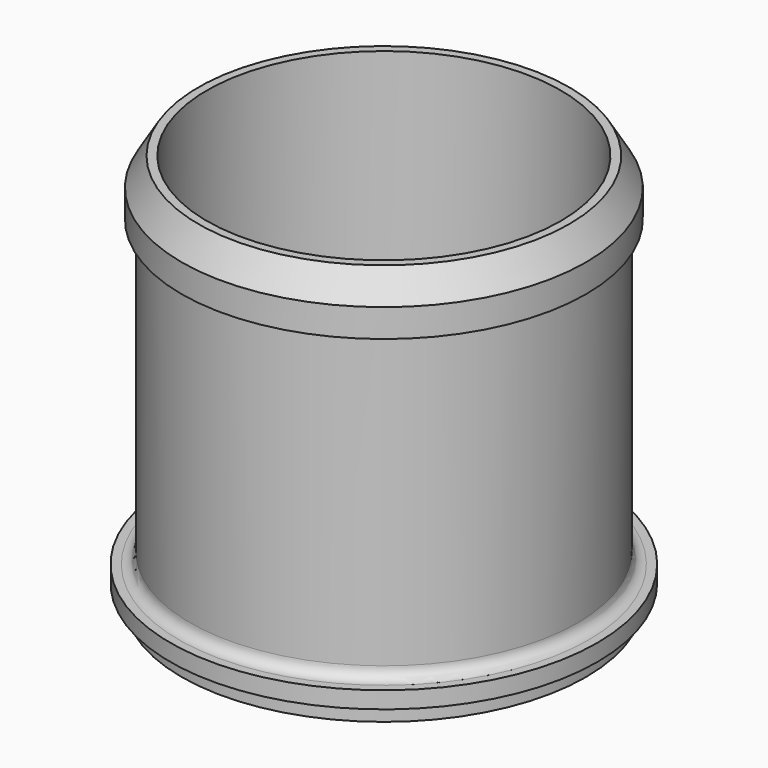
from build123d import *

# Parameters (mm, degrees)
F2_SIZE2 = 3
F2_SIZE  = 5
F3_R     = 2


# Not quite as in the source:
# - a fillet or chamfer that OpenCascade refuses, or shapes differently, is made with other operations: its cross-section is extruded or revolved along the edge and cut away or added


with BuildPart() as f1:
    # F0 (on Front) → F1 (revolve)
    with BuildSketch(Plane.XZ):
        Polygon((34.5, 70), (31.5, 70), (31.5, 0), (36, 0), (36, 3), (38, 3), (38, 6), (34.5, 6), (34.5, 60), (36, 60), (36, 70), align=None)
    revolve(axis=Axis((0, 0, 35), (0, 0, 1)))

    # F2
    f2_edges = [f1.edges().sort_by_distance(p)[0] for p in [
        (-36, 0, 70),
    ]]
    f2_side = f1.faces().sort_by_distance((-36, 0, 65))[0]
    chamfer(f2_edges, length=F2_SIZE, length2=F2_SIZE2, reference=f2_side)

    # F3
    f3_edges = [f1.edges().sort_by_distance(p)[0] for p in [
        (-34.5, 0, 6),
    ]]
    fillet(f3_edges, radius=F3_R)

    # F4: fillet of radius 5 on 1 edges, made by hand

    # F4_s1 → F4_t2 (revolve, cut)
    with BuildSketch(Plane.XZ):
        with BuildLine():
            ThreePointArc((31.5, 4.9749371855), (32.7919007565, 1.6208352193), (36, 0))
            Line((36, 0), (31.5, 0))
            Line((31.5, 0), (31.5, 4.9749371855))
        make_face()
    revolve(axis=Axis((0, 0, 0), (0, 0, 1)), mode=Mode.SUBTRACT)


solid = f1.part
